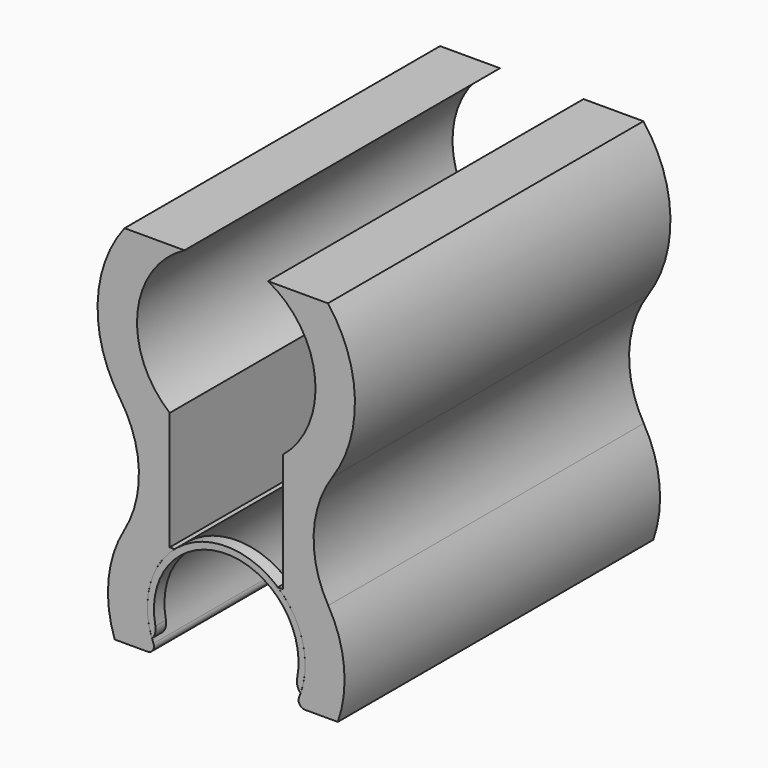
from build123d import *

# Parameters (mm, degrees)
F1_DEPTH      = 30
F3_DEPTH      = 27
F5_DEPTH      = 1
F7_DEPTH      = 1
F8_T1_DEPTH   = 5.7000067135
F8_2_T1_DEPTH = 5.7000067135
F9_R          = 0.5


# Not quite as in the source:
# - a fillet or chamfer that OpenCascade refuses, or shapes differently, is made with other operations: its cross-section is extruded or revolved along the edge and cut away or added


with BuildPart() as f1:
    # F0 (on Front) → F1 (new body)
    with BuildSketch(Plane.XZ):
        with BuildLine():
            ThreePointArc((3.1776069014, 15.7894908219), (0, 3), (-3.1776069014, 15.7894908219))
            Line((-3.1776069014, 15.7894908219), (-7.7352524556, 15.7894908219))
            ThreePointArc((-7.7352524556, 15.7894908219), (-9.7854255442, 10.0715856127), (-8.0680556753, 4.245069466))
            ThreePointArc((-8.0680556753, 4.245069466), (-6.6495163105, -0.0531637642), (-7.7599288431, -4.4411071136))
            ThreePointArc((-7.7599288431, -4.4411071136), (-8.9588464195, -8.1403077112), (-8.4852813742, -12))
            Line((-8.4852813742, -12), (-5.1961524227, -12))
            ThreePointArc((-5.1961524227, -12), (0, -3), (5.1961524227, -12))
            Line((5.1961524227, -12), (8.4852813742, -12))
            ThreePointArc((8.4852813742, -12), (8.9588464195, -8.1403077112), (7.7599288431, -4.4411071136))
            ThreePointArc((7.7599288431, -4.4411071136), (6.6495163105, -0.0531637642), (8.0680556753, 4.245069466))
            ThreePointArc((8.0680556753, 4.245069466), (9.7854255442, 10.0715856127), (7.7352524556, 15.7894908219))
            Line((7.7352524556, 15.7894908219), (3.1776069014, 15.7894908219))
        make_face()
    extrude(amount=F1_DEPTH)

    # F2 (on face) → F3 (cut)
    with BuildSketch(Plane.XZ.offset(30)):
        with BuildLine():
            ThreePointArc((4.3, 4.535236772), (0, 3), (-4.3, 4.535236772))
            Line((-4.3, 4.535236772), (-4.3, -4.464763228))
            Line((-4.3, -4.464763228), (4.3, -4.464763228))
            Line((4.3, -4.464763228), (4.3, 4.535236772))
        make_face()
    extrude(amount=-F3_DEPTH, mode=Mode.SUBTRACT)

    # F9
    f9_edges = [f1.edges().sort_by_distance(p)[0] for p in [
        (5.196152, -15, -12),
        (-5.196152, -15, -12),
    ]]
    fillet(f9_edges, radius=F9_R)


with BuildPart() as f5:
    # F4 (on face) → F5 (new body)
    with BuildSketch(Plane.XZ.offset(30)):
        with BuildLine():
            Line((5.123475383, -11), (5.6568542495, -11))
            ThreePointArc((5.6568542495, -11), (0, -3), (-5.6568542495, -11))
            Line((-5.6568542495, -11), (-5.123475383, -11))
            ThreePointArc((-5.123475383, -11), (0, -3.5), (5.123475383, -11))
        make_face()
    extrude(amount=-F5_DEPTH)

    # F8: fillet of radius 1 on 2 edges, made by hand

    # F8_s2 → F8_t1 (cut)
    with BuildSketch(Plane.XZ.offset(26.6499966433)):
        with BuildLine():
            ThreePointArc((5.3892153407, -10.0983433031), (5.4104140841, -10.5826008761), (5.6568542495, -11))
            Line((5.6568542495, -11), (5.123475383, -11))
            ThreePointArc((5.123475383, -11), (5.2756433506, -10.5548592339), (5.3892153407, -10.0983433031))
        make_face()
        with BuildLine():
            ThreePointArc((-5.3892153407, -10.0983433031), (-5.4104140841, -10.5826008761), (-5.6568542495, -11))
            Line((-5.6568542495, -11), (-5.123475383, -11))
            ThreePointArc((-5.123475383, -11), (-5.2756433506, -10.5548592339), (-5.3892153407, -10.0983433031))
        make_face()
    extrude(amount=F8_T1_DEPTH, mode=Mode.SUBTRACT)


with BuildPart() as f7:
    # F6 (on face) → F7 (new body)
    with BuildSketch(Plane(origin=(0, 0, 0), x_dir=(-1, 0, 0), z_dir=(0, 1, 0))):
        with BuildLine():
            ThreePointArc((5.6568542495, -11), (0, -3), (-5.6568542495, -11))
            Line((-5.6568542495, -11), (-5.123475383, -11))
            ThreePointArc((-5.123475383, -11), (0, -3.5), (5.123475383, -11))
            Line((5.123475383, -11), (5.6568542495, -11))
        make_face()
    extrude(amount=-F7_DEPTH)

    # F8#2: fillet of radius 1 on 2 edges, made by hand

    # F8_2_s2 → F8_2_t1 (cut)
    with BuildSketch(Plane.XZ.offset(-2.3500033567)):
        with BuildLine():
            ThreePointArc((5.6568542495, -11), (5.4104140841, -10.5826008761), (5.3892153407, -10.0983433031))
            ThreePointArc((5.3892153407, -10.0983433031), (5.2756433506, -10.5548592339), (5.123475383, -11))
            Line((5.123475383, -11), (5.6568542495, -11))
        make_face()
        with BuildLine():
            ThreePointArc((-5.3892153407, -10.0983433031), (-5.4104140841, -10.5826008761), (-5.6568542495, -11))
            Line((-5.6568542495, -11), (-5.123475383, -11))
            ThreePointArc((-5.123475383, -11), (-5.2756433506, -10.5548592339), (-5.3892153407, -10.0983433031))
        make_face()
    extrude(amount=F8_2_T1_DEPTH, mode=Mode.SUBTRACT)


solid = Compound([f1.part, f5.part, f7.part])
